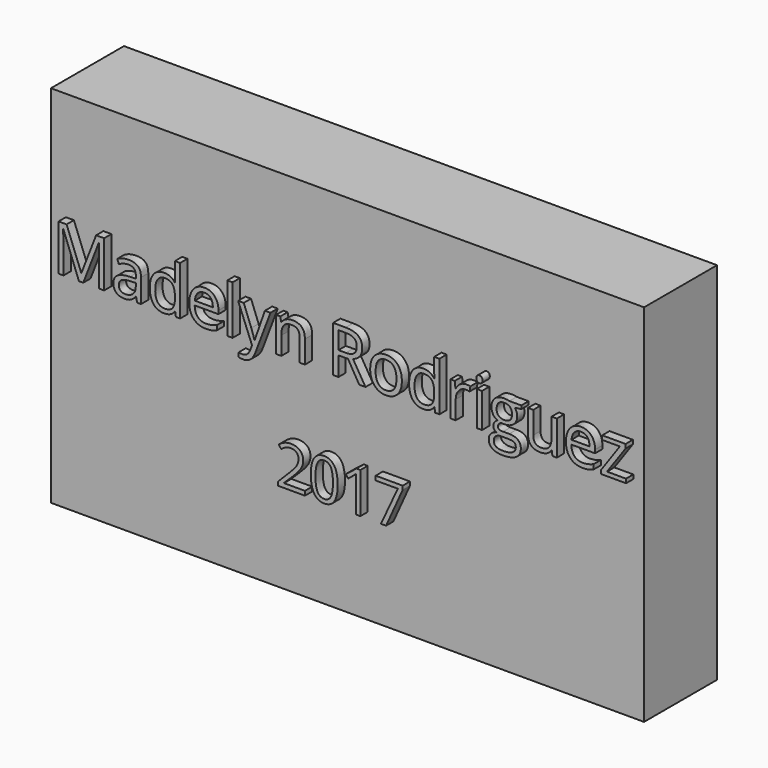
from build123d import *

# Parameters (mm, degrees)
F0_W         = 165.1
F0_H         = 101.6
F1_DEPTH     = 25.4
F2_TEXT_SIZE = 17.9247536127
F3_DEPTH     = 2.54
F4_TEXT_SIZE = 15.8404789141
F5_DEPTH     = 2.54


# Not quite as in the source:
# - Text() gives the source's letters only with a copy of the font that has no kerning and outlines rounded to 1/6400 em; it was checked with that copy


with BuildPart() as f1:
    # F0 (on Front) → F1 (new body)
    with BuildSketch(Plane.XZ):
        Rectangle(F0_W, F0_H)
    extrude(amount=F1_DEPTH)

    # F2 (on face) → F3 (join)
    with BuildSketch(Plane.XZ.offset(25.4)):
        with Locations((-80.1519602537, 7.7452617697)):
            Text('Madelyn Rodriguez', F2_TEXT_SIZE, font='Open Sans', text_align=(TextAlign.LEFT, TextAlign.BOTTOM))
    extrude(amount=F3_DEPTH)

    # F4 (on face) → F5 (join)
    with BuildSketch(Plane.XZ.offset(25.4)):
        with Locations((-18.0239267647, -24.369224906)):
            Text('2017', F4_TEXT_SIZE, font='Open Sans', text_align=(TextAlign.LEFT, TextAlign.BOTTOM))
    extrude(amount=F5_DEPTH)


solid = f1.part
